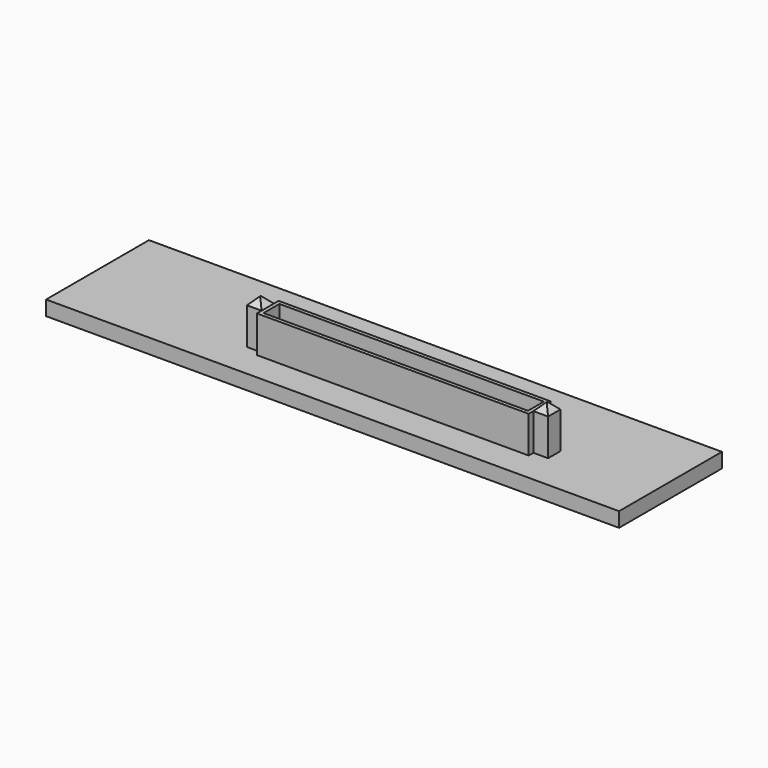
from build123d import *

# Parameters (mm, degrees)
F0_W     = 78
F0_H     = 17.5
F1_DEPTH = 2
F2_W     = 36
F2_H     = 2.7
F2_W_2   = 2
F2_H_2   = 2.1
F3_DEPTH = 5
F4_W     = 2
F4_H     = 2.1
F5_DEPTH = 1
F6_SIZE  = 0.99999


# Not quite as in the source:
# - a fillet or chamfer is up to 0.001 mm smaller than in the source, because OpenCascade refuses the exact size


with BuildPart() as f1:
    # F0 (on Top) → F1 (new body)
    with BuildSketch(Plane.XY):
        Rectangle(F0_W, F0_H)
    extrude(amount=F1_DEPTH)

    # F2 (on face) → F3 (join)
    with BuildSketch(Plane.XY.offset(2)):
        Polygon((-13.5, -3.95), (-13.5, -4.75), (23.5, -4.75), (23.5, -3.95), (23.5, -1.85), (23.5, -1.05), (-13.5, -1.05), (-13.5, -1.85), align=None)
        with Locations((5, -2.9)):
            Rectangle(F2_W, F2_H, mode=Mode.SUBTRACT)
        with Locations((-14.5, -2.9)):
            Rectangle(F2_W_2, F2_H_2)
        with Locations((24.5, -2.9)):
            Rectangle(F2_W_2, F2_H_2)
    extrude(amount=F3_DEPTH)

    # F4 (on face) → F5 (join)
    with BuildSketch(Plane.XY.offset(7)):
        with Locations((-14.5, -2.9)):
            Rectangle(F4_W, F4_H)
        with Locations((24.5, -2.9)):
            Rectangle(F4_W, F4_H)
    extrude(amount=F5_DEPTH)

    # F6 (size 1 in the source; OpenCascade refuses exactly that, so slightly less here)
    f6_edges = [f1.edges().sort_by_distance(p)[0] for p in [
        (-15.5, -2.9, 8),
        (-14.5, -1.85, 8),
        (-13.5, -2.9, 8),
        (-14.5, -3.95, 8),
        (24.5, -1.85, 8),
        (23.5, -2.9, 8),
        (25.5, -2.9, 8),
        (24.5, -3.95, 8),
    ]]
    chamfer(f6_edges, length=F6_SIZE)


solid = f1.part
